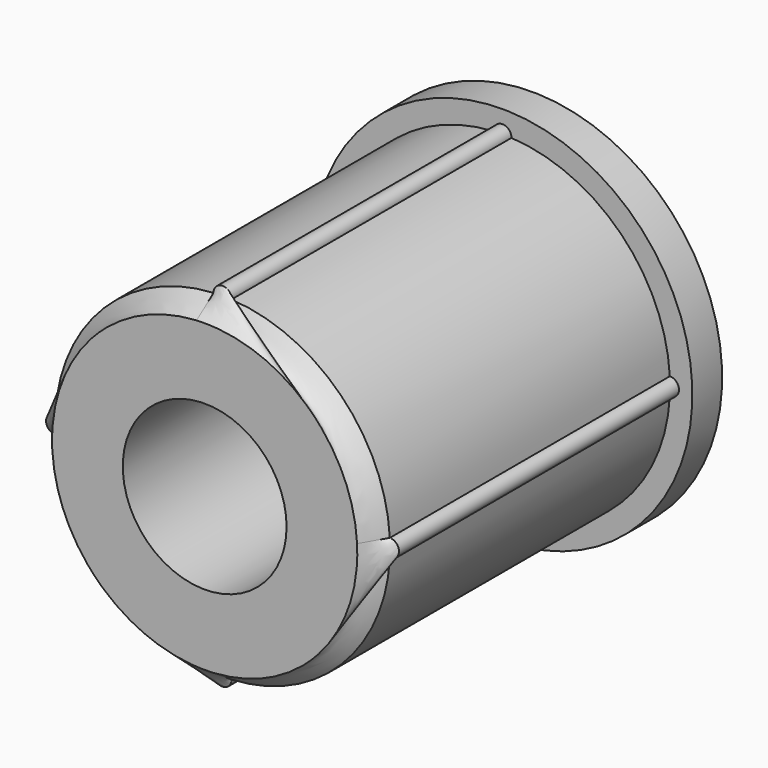
from build123d import *

# Parameters (mm, degrees)
F1_DEPTH       = 23.5
F5_R           = 12.75
F6_DEPTH       = 2.5
F8_D           = 5.9
F8_CSINK_D     = 6.8
F8_CSINK_ANGLE = 90
F9_R           = 5.5
F10_DEPTH      = 17.5


# Not quite as in the source:
# - the arcs of a loft's sections are written as splines that run evenly, so that the points pair up as in the source's solid


with BuildPart() as f1:
    # F0 (on Front) → F1 (new body)
    with BuildSketch(Plane.XZ):
        with BuildLine():
            ThreePointArc((0.5997866287, 11.234), (0, 11.85), (-0.5997866287, 11.234))
            ThreePointArc((-0.5997866287, 11.234), (-7.9549512883, 7.9549512883), (-11.234, 0.5997866287))
            ThreePointArc((-11.234, 0.5997866287), (-11.85, 0), (-11.234, -0.5997866287))
            ThreePointArc((-11.234, -0.5997866287), (-7.9549512883, -7.9549512883), (-0.5997866287, -11.234))
            ThreePointArc((-0.5997866287, -11.234), (0, -11.85), (0.5997866287, -11.234))
            ThreePointArc((0.5997866287, -11.234), (7.9549512883, -7.9549512883), (11.234, -0.5997866287))
            ThreePointArc((11.234, -0.5997866287), (11.85, 0), (11.234, 0.5997866287))
            ThreePointArc((11.234, 0.5997866287), (7.9549512883, 7.9549512883), (0.5997866287, 11.234))
        make_face()
    extrude(amount=F1_DEPTH)

    # F1_face (on face) → F4 section 0
    with BuildSketch(Plane.XZ.offset(23.5)):
        with BuildLine():
            add(Edge.make_bspline(
                [(0.5997866287, 11.234), (0.6016799219, 11.3049732474), (0.5908445992, 11.376267359), (0.5450568557, 11.5106795168), (0.5101164815, 11.5737621993), (0.4204642218, 11.6838785828), (0.3657759235, 11.7308833124), (0.2434389451, 11.8029722112), (0.1758224517, 11.8280374139), (0.0360563953, 11.853109213), (-0.0360563953, 11.853109213), (-0.1758224517, 11.8280374139), (-0.2434389451, 11.8029722112), (-0.3657759235, 11.7308833124), (-0.4204642218, 11.6838785828), (-0.5101164815, 11.5737621993), (-0.5450568557, 11.5106795168), (-0.5908445992, 11.376267359), (-0.6016799219, 11.3049732474), (-0.5997866287, 11.234)],
                knots=[0, 0, 0, 0, 0.1111111111, 0.1111111111, 0.2222222222, 0.2222222222, 0.3333333333, 0.3333333333, 0.4444444444, 0.4444444444, 0.5555555556, 0.5555555556, 0.6666666667, 0.6666666667, 0.7777777778, 0.7777777778, 0.8888888889, 0.8888888889, 1, 1, 1, 1], degree=3))
            add(Edge.make_bspline(
                [(-0.5997866287, 11.234), (-1.9704441734, 11.1608201827), (-3.3271537618, 10.8340484232), (-5.834489174, 9.7162386482), (-6.984369661, 8.9255329157), (-8.9255329157, 6.984369661), (-9.7162386482, 5.834489174), (-10.8340484232, 3.3271537618), (-11.1608201827, 1.9704441734), (-11.234, 0.5997866287)],
                knots=[0, 0, 0, 0, 0.25, 0.25, 0.5, 0.5, 0.75, 0.75, 1, 1, 1, 1], degree=3))
            add(Edge.make_bspline(
                [(-11.234, 0.5997866287), (-11.3049732474, 0.6016799219), (-11.376267359, 0.5908445992), (-11.5106795168, 0.5450568557), (-11.5737621993, 0.5101164815), (-11.6838785828, 0.4204642218), (-11.7308833124, 0.3657759235), (-11.8029722112, 0.2434389451), (-11.8280374139, 0.1758224517), (-11.853109213, 0.0360563953), (-11.853109213, -0.0360563953), (-11.8280374139, -0.1758224517), (-11.8029722112, -0.2434389451), (-11.7308833124, -0.3657759235), (-11.6838785828, -0.4204642218), (-11.5737621993, -0.5101164815), (-11.5106795168, -0.5450568557), (-11.376267359, -0.5908445992), (-11.3049732474, -0.6016799219), (-11.234, -0.5997866287)],
                knots=[0, 0, 0, 0, 0.1111111111, 0.1111111111, 0.2222222222, 0.2222222222, 0.3333333333, 0.3333333333, 0.4444444444, 0.4444444444, 0.5555555556, 0.5555555556, 0.6666666667, 0.6666666667, 0.7777777778, 0.7777777778, 0.8888888889, 0.8888888889, 1, 1, 1, 1], degree=3))
            add(Edge.make_bspline(
                [(-11.234, -0.5997866287), (-11.1608201827, -1.9704441734), (-10.8340484232, -3.3271537618), (-9.7162386482, -5.834489174), (-8.9255329157, -6.984369661), (-6.984369661, -8.9255329157), (-5.834489174, -9.7162386482), (-3.3271537618, -10.8340484232), (-1.9704441734, -11.1608201827), (-0.5997866287, -11.234)],
                knots=[0, 0, 0, 0, 0.25, 0.25, 0.5, 0.5, 0.75, 0.75, 1, 1, 1, 1], degree=3))
            add(Edge.make_bspline(
                [(-0.5997866287, -11.234), (-0.6016799219, -11.3049732474), (-0.5908445992, -11.376267359), (-0.5450568557, -11.5106795168), (-0.5101164815, -11.5737621993), (-0.4204642218, -11.6838785828), (-0.3657759235, -11.7308833124), (-0.2434389451, -11.8029722112), (-0.1758224517, -11.8280374139), (-0.0360563953, -11.853109213), (0.0360563953, -11.853109213), (0.1758224517, -11.8280374139), (0.2434389451, -11.8029722112), (0.3657759235, -11.7308833124), (0.4204642218, -11.6838785828), (0.5101164815, -11.5737621993), (0.5450568557, -11.5106795168), (0.5908445992, -11.376267359), (0.6016799219, -11.3049732474), (0.5997866287, -11.234)],
                knots=[0, 0, 0, 0, 0.1111111111, 0.1111111111, 0.2222222222, 0.2222222222, 0.3333333333, 0.3333333333, 0.4444444444, 0.4444444444, 0.5555555556, 0.5555555556, 0.6666666667, 0.6666666667, 0.7777777778, 0.7777777778, 0.8888888889, 0.8888888889, 1, 1, 1, 1], degree=3))
            add(Edge.make_bspline(
                [(0.5997866287, -11.234), (1.9704441734, -11.1608201827), (3.3271537618, -10.8340484232), (5.834489174, -9.7162386482), (6.984369661, -8.9255329157), (8.9255329157, -6.984369661), (9.7162386482, -5.834489174), (10.8340484232, -3.3271537618), (11.1608201827, -1.9704441734), (11.234, -0.5997866287)],
                knots=[0, 0, 0, 0, 0.25, 0.25, 0.5, 0.5, 0.75, 0.75, 1, 1, 1, 1], degree=3))
            add(Edge.make_bspline(
                [(11.234, -0.5997866287), (11.3049732474, -0.6016799219), (11.376267359, -0.5908445992), (11.5106795168, -0.5450568557), (11.5737621993, -0.5101164815), (11.6838785828, -0.4204642218), (11.7308833124, -0.3657759235), (11.8029722112, -0.2434389451), (11.8280374139, -0.1758224517), (11.853109213, -0.0360563953), (11.853109213, 0.0360563953), (11.8280374139, 0.1758224517), (11.8029722112, 0.2434389451), (11.7308833124, 0.3657759235), (11.6838785828, 0.4204642218), (11.5737621993, 0.5101164815), (11.5106795168, 0.5450568557), (11.376267359, 0.5908445992), (11.3049732474, 0.6016799219), (11.234, 0.5997866287)],
                knots=[0, 0, 0, 0, 0.1111111111, 0.1111111111, 0.2222222222, 0.2222222222, 0.3333333333, 0.3333333333, 0.4444444444, 0.4444444444, 0.5555555556, 0.5555555556, 0.6666666667, 0.6666666667, 0.7777777778, 0.7777777778, 0.8888888889, 0.8888888889, 1, 1, 1, 1], degree=3))
            add(Edge.make_bspline(
                [(11.234, 0.5997866287), (11.1608201827, 1.9704441734), (10.8340484232, 3.3271537618), (9.7162386482, 5.834489174), (8.9255329157, 6.984369661), (6.984369661, 8.9255329157), (5.834489174, 9.7162386482), (3.3271537618, 10.8340484232), (1.9704441734, 11.1608201827), (0.5997866287, 11.234)],
                knots=[0, 0, 0, 0, 0.25, 0.25, 0.5, 0.5, 0.75, 0.75, 1, 1, 1, 1], degree=3))
        make_face()
    # F3 (on offset) → F4 section 1
    with BuildSketch(Plane.XZ.offset(25)):
        with BuildLine():
            add(Edge.make_bspline(
                [(-0.5464722617, 10.2354222222), (-1.8862858976, 10.1638891704), (-3.2113491637, 9.8259836202), (-5.6322529271, 8.6683588136), (-6.7271409022, 7.8490950331), (-7.6239507036, 6.8511222196)],
                knots=[0, 0, 0, 0, 0.5, 0.5, 1, 1, 1, 1], degree=3))
            add(Edge.make_bspline(
                [(-7.6239507036, 6.8511222196), (-8.5207605051, 5.8531494062), (-9.2187864201, 4.6772528793), (-10.112059537, 2.1468510607), (-10.306955274, 0.7933413741), (-10.2354222222, -0.5464722617)],
                knots=[0, 0, 0, 0, 0.5, 0.5, 1, 1, 1, 1], degree=3))
            add(Edge.make_bspline(
                [(-10.2354222222, -0.5464722617), (-10.1638891704, -1.8862858976), (-9.8259836202, -3.2113491637), (-8.6683588136, -5.6322529271), (-7.8490950331, -6.7271409022), (-6.8511222196, -7.6239507036)],
                knots=[0, 0, 0, 0, 0.5, 0.5, 1, 1, 1, 1], degree=3))
            add(Edge.make_bspline(
                [(-6.8511222196, -7.6239507036), (-5.8531494062, -8.5207605051), (-4.6772528793, -9.2187864201), (-2.1468510607, -10.112059537), (-0.7933413741, -10.306955274), (0.5464722617, -10.2354222222)],
                knots=[0, 0, 0, 0, 0.5, 0.5, 1, 1, 1, 1], degree=3))
            add(Edge.make_bspline(
                [(0.5464722617, -10.2354222222), (1.8862858976, -10.1638891704), (3.2113491637, -9.8259836202), (5.6322529271, -8.6683588136), (6.7271409022, -7.8490950331), (7.6239507036, -6.8511222196)],
                knots=[0, 0, 0, 0, 0.5, 0.5, 1, 1, 1, 1], degree=3))
            add(Edge.make_bspline(
                [(7.6239507036, -6.8511222196), (8.5207605051, -5.8531494062), (9.2187864201, -4.6772528793), (10.112059537, -2.1468510607), (10.306955274, -0.7933413741), (10.2354222222, 0.5464722617)],
                knots=[0, 0, 0, 0, 0.5, 0.5, 1, 1, 1, 1], degree=3))
            add(Edge.make_bspline(
                [(10.2354222222, 0.5464722617), (10.1638891704, 1.8862858976), (9.8259836202, 3.2113491637), (8.6683588136, 5.6322529271), (7.8490950331, 6.7271409022), (6.8511222196, 7.6239507036)],
                knots=[0, 0, 0, 0, 0.5, 0.5, 1, 1, 1, 1], degree=3))
            add(Edge.make_bspline(
                [(6.8511222196, 7.6239507036), (5.8531494062, 8.5207605051), (4.6772528793, 9.2187864201), (2.1468510607, 10.112059537), (0.7933413741, 10.306955274), (-0.5464722617, 10.2354222222)],
                knots=[0, 0, 0, 0, 0.5, 0.5, 1, 1, 1, 1], degree=3))
        make_face()
    loft(ruled=True)

    # F5 (on face) → F6 (join)
    with BuildSketch(Plane(origin=(0, 0, 0), x_dir=(-1, 0, 0), z_dir=(0, 1, 0))):
        Circle(F5_R)
    extrude(amount=F6_DEPTH)

    # F8 (through all)
    with Locations(Plane(origin=(0, 2.5, 0), x_dir=(-1, 0, 0), z_dir=(0, 1, 0))):
        with Locations((0, 0)):
            CounterSinkHole(F8_D / 2, F8_CSINK_D / 2, counter_sink_angle=F8_CSINK_ANGLE)

    # F9 (on face) → F10 (cut)
    with BuildSketch(Plane.XZ.offset(25)):
        Circle(F9_R)
    extrude(amount=-F10_DEPTH, mode=Mode.SUBTRACT)


solid = f1.part
